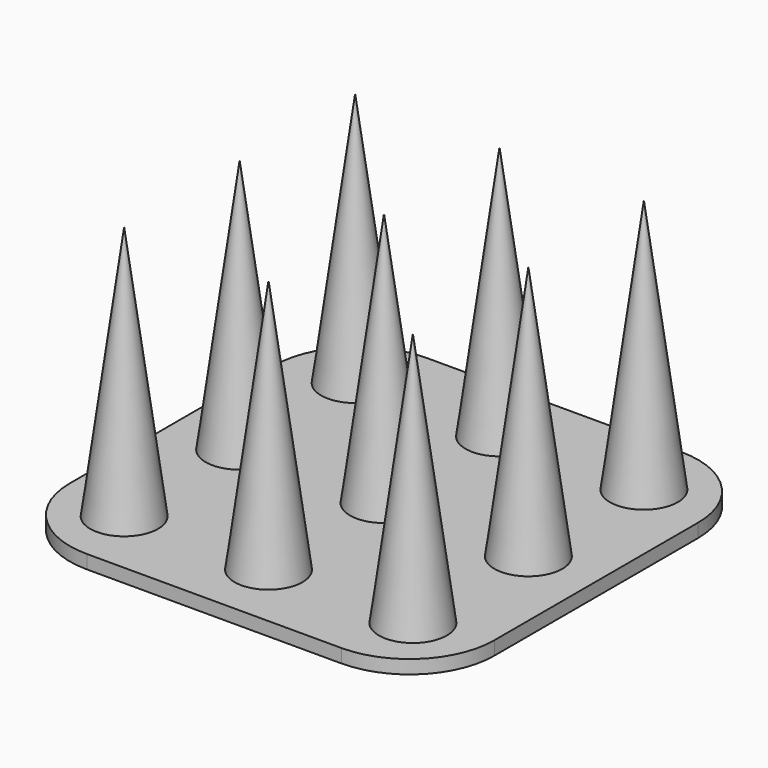
from build123d import *

# Parameters (mm, degrees)
F1_DEPTH   = 0.8
F2_R       = 2
F3_DEPTH   = 15
F4_SIZE2   = 14.99999
F4_SIZE    = 1.99999
F4_2_SIZE2 = 14.99999
F4_2_SIZE  = 1.99999
F4_3_SIZE2 = 14.99999
F4_3_SIZE  = 1.99999
F4_4_SIZE2 = 14.99999
F4_4_SIZE  = 1.99999
F4_5_SIZE2 = 14.99999
F4_5_SIZE  = 1.99999
F4_6_SIZE2 = 14.99999
F4_6_SIZE  = 1.99999
F4_7_SIZE2 = 14.99999
F4_7_SIZE  = 1.99999
F4_8_SIZE2 = 14.99999
F4_8_SIZE  = 1.99999
F4_9_SIZE2 = 14.99999
F4_9_SIZE  = 1.99999


# Not quite as in the source:
# - a fillet or chamfer is up to 0.001 mm smaller than in the source, because OpenCascade refuses the exact size


with BuildPart() as f1:
    # F0 (on Top) → F1 (new body)
    with BuildSketch(Plane.XY):
        with BuildLine():
            ThreePointArc((-12.5, -7.5), (-11.0355339059, -11.0355339059), (-7.5, -12.5))
            Line((-7.5, -12.5), (7.5, -12.5))
            ThreePointArc((7.5, -12.5), (11.0355339059, -11.0355339059), (12.5, -7.5))
            Line((12.5, -7.5), (12.5, 7.5))
            ThreePointArc((12.5, 7.5), (11.0355339059, 11.0355339059), (7.5, 12.5))
            Line((7.5, 12.5), (-7.5, 12.5))
            ThreePointArc((-7.5, 12.5), (-11.0355339059, 11.0355339059), (-12.5, 7.5))
            Line((-12.5, 7.5), (-12.5, -7.5))
        make_face()
    extrude(amount=F1_DEPTH)

    # F2 (on face) → F3 (join)
    with BuildSketch(Plane.XY.offset(0.8)):
        with Locations((-8.5, -8.5)):
            Circle(F2_R)
        with Locations((-8.5, 0)):
            Circle(F2_R)
        with Locations((-8.5, 8.5)):
            Circle(F2_R)
        with Locations((0, -8.5)):
            Circle(F2_R)
        Circle(F2_R)
        with Locations((0, 8.5)):
            Circle(F2_R)
        with Locations((8.5, -8.5)):
            Circle(F2_R)
        with Locations((8.5, 0)):
            Circle(F2_R)
        with Locations((8.5, 8.5)):
            Circle(F2_R)
    extrude(amount=F3_DEPTH)

    # F4 (size 2 and 15 in the source; OpenCascade refuses exactly that, so slightly less here)
    f4_edges = [f1.edges().sort_by_distance(p)[0] for p in [
        (-10.5, -8.5, 15.8),
    ]]
    f4_side = f1.faces().sort_by_distance((-8.5, -8.5, 15.8))[0]
    chamfer(f4_edges, length=F4_SIZE, length2=F4_SIZE2, reference=f4_side)

    # F4#2 (size 2 and 15 in the source; OpenCascade refuses exactly that, so slightly less here)
    f4_2_edges = [f1.edges().sort_by_distance(p)[0] for p in [
        (-10.5, 0, 15.8),
    ]]
    f4_2_side = f1.faces().sort_by_distance((-8.5, 0, 15.8))[0]
    chamfer(f4_2_edges, length=F4_2_SIZE, length2=F4_2_SIZE2, reference=f4_2_side)

    # F4#3 (size 2 and 15 in the source; OpenCascade refuses exactly that, so slightly less here)
    f4_3_edges = [f1.edges().sort_by_distance(p)[0] for p in [
        (-10.5, 8.5, 15.8),
    ]]
    f4_3_side = f1.faces().sort_by_distance((-8.5, 8.5, 15.8))[0]
    chamfer(f4_3_edges, length=F4_3_SIZE, length2=F4_3_SIZE2, reference=f4_3_side)

    # F4#4 (size 2 and 15 in the source; OpenCascade refuses exactly that, so slightly less here)
    f4_4_edges = [f1.edges().sort_by_distance(p)[0] for p in [
        (-2, 8.5, 15.8),
    ]]
    f4_4_side = f1.faces().sort_by_distance((0, 8.5, 15.8))[0]
    chamfer(f4_4_edges, length=F4_4_SIZE, length2=F4_4_SIZE2, reference=f4_4_side)

    # F4#5 (size 2 and 15 in the source; OpenCascade refuses exactly that, so slightly less here)
    f4_5_edges = [f1.edges().sort_by_distance(p)[0] for p in [
        (-2, 0, 15.8),
    ]]
    f4_5_side = f1.faces().sort_by_distance((0, 0, 15.8))[0]
    chamfer(f4_5_edges, length=F4_5_SIZE, length2=F4_5_SIZE2, reference=f4_5_side)

    # F4#6 (size 2 and 15 in the source; OpenCascade refuses exactly that, so slightly less here)
    f4_6_edges = [f1.edges().sort_by_distance(p)[0] for p in [
        (-2, -8.5, 15.8),
    ]]
    f4_6_side = f1.faces().sort_by_distance((0, -8.5, 15.8))[0]
    chamfer(f4_6_edges, length=F4_6_SIZE, length2=F4_6_SIZE2, reference=f4_6_side)

    # F4#7 (size 2 and 15 in the source; OpenCascade refuses exactly that, so slightly less here)
    f4_7_edges = [f1.edges().sort_by_distance(p)[0] for p in [
        (6.5, -8.5, 15.8),
    ]]
    f4_7_side = f1.faces().sort_by_distance((8.5, -8.5, 15.8))[0]
    chamfer(f4_7_edges, length=F4_7_SIZE, length2=F4_7_SIZE2, reference=f4_7_side)

    # F4#8 (size 2 and 15 in the source; OpenCascade refuses exactly that, so slightly less here)
    f4_8_edges = [f1.edges().sort_by_distance(p)[0] for p in [
        (6.5, 0, 15.8),
    ]]
    f4_8_side = f1.faces().sort_by_distance((8.5, 0, 15.8))[0]
    chamfer(f4_8_edges, length=F4_8_SIZE, length2=F4_8_SIZE2, reference=f4_8_side)

    # F4#9 (size 2 and 15 in the source; OpenCascade refuses exactly that, so slightly less here)
    f4_9_edges = [f1.edges().sort_by_distance(p)[0] for p in [
        (6.5, 8.5, 15.8),
    ]]
    f4_9_side = f1.faces().sort_by_distance((8.5, 8.5, 15.8))[0]
    chamfer(f4_9_edges, length=F4_9_SIZE, length2=F4_9_SIZE2, reference=f4_9_side)


solid = f1.part
